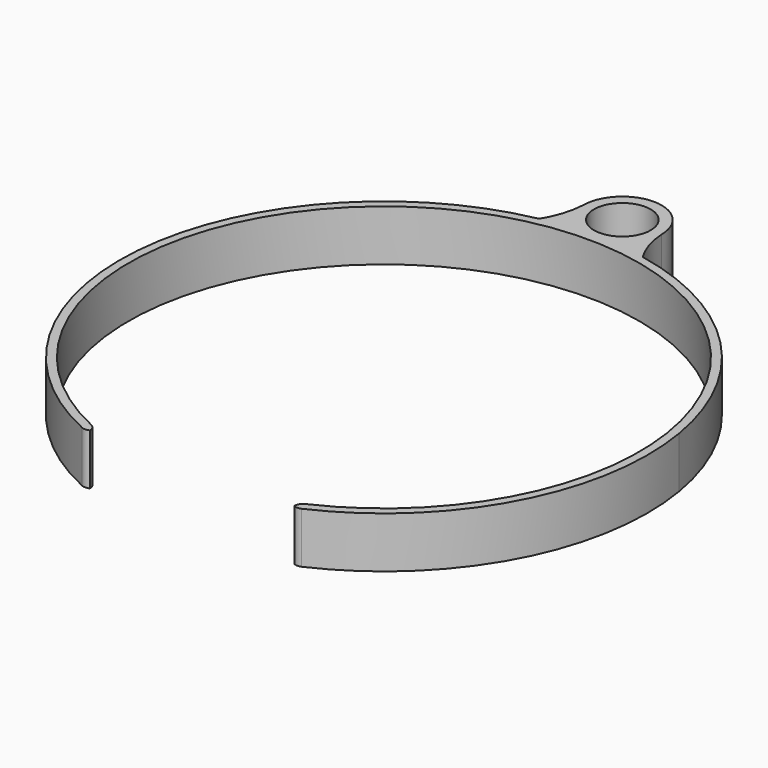
from build123d import *

# Parameters (mm, degrees)
F0_R         = 46.5
F0_R_2       = 45
F1_DEPTH     = 9
F3_DEPTH     = 25
F5_DEPTH     = 25
F7_DEPTH     = 9
F9_DEPTH     = 9
F11_DEPTH    = 9
F13_DEPTH    = 25
F15_DEPTH    = 25
F16_R        = 45
F17_DEPTH    = 9
F18_R        = 45
F19_DEPTH    = 25
F21_DEPTH    = 25
F22_R        = 1.55
F23_T1_DEPTH = 16.2900218994
F24_T1_DEPTH = 16.2900218994


# Not quite as in the source:
# - a fillet or chamfer that OpenCascade refuses, or shapes differently, is made with other operations: its cross-section is extruded or revolved along the edge and cut away or added


with BuildPart() as f1:
    # F0 (on Top) → F1 (new body)
    with BuildSketch(Plane.XY):
        Circle(F0_R)
        Circle(F0_R_2, mode=Mode.SUBTRACT)
    extrude(amount=F1_DEPTH)

    # F2 (on face) → F3 (cut)
    with BuildSketch(Plane.XY.offset(9)):
        Polygon((64.8135244846, -21.5104352683), (0, -21.5104352683), (-51.5724048018, -21.5104352683), (-51.5724048018, -59.9158406258), (64.033716917, -57.7713772655), align=None)
    extrude(amount=-F3_DEPTH, mode=Mode.SUBTRACT)

    # F4 (on face) → F5 (cut)
    with BuildSketch(Plane.XY.offset(9)):
        with BuildLine():
            ThreePointArc((-40.5525222975, -19.506228116), (-40.9032938672, -20.5072072896), (-41.9042730407, -20.1564357199))
            Line((-41.9042730407, -20.1564357199), (-43.4346050024, -22.7221362293))
            Line((-43.4346050024, -22.7221362293), (-36.3525599241, -23.4547629952))
            Line((-36.3525599241, -23.4547629952), (-40.5525222975, -19.506228116))
        make_face()
        with BuildLine():
            Line((43.4346050024, -22.7221362293), (41.9042730407, -20.1564357199))
            ThreePointArc((41.9042730407, -20.1564357199), (40.9032938672, -20.5072072896), (40.5525222975, -19.506228116))
            Line((40.5525222975, -19.506228116), (36.3525599241, -23.4547629952))
            Line((36.3525599241, -23.4547629952), (43.4346050024, -22.7221362293))
        make_face()
    extrude(amount=-F5_DEPTH, mode=Mode.SUBTRACT)

    # F6 (on face) → F7 (join)
    with BuildSketch(Plane.XY.offset(9)):
        with BuildLine():
            ThreePointArc((6.9320949163, 52.5), (-4.9017313232, 57.4017313232), (0, 45.5679050837))
            ThreePointArc((0, 45.5679050837), (4.9017313232, 47.5982686768), (6.9320949163, 52.5))
        make_face()
        with BuildLine():
            ThreePointArc((5, 52.5), (3.5355339059, 48.9644660941), (0, 47.5))
            ThreePointArc((0, 47.5), (-3.5355339059, 56.0355339059), (5, 52.5))
        make_face(mode=Mode.SUBTRACT)
    extrude(amount=-F7_DEPTH)

    # F8 (on face) → F9 (join)
    with BuildSketch(Plane.XY.offset(9)):
        with BuildLine():
            ThreePointArc((-6.9320949163, 52.5), (-7.6007884485, 48.9142518774), (-9.1181185374, 45.5972577502))
            ThreePointArc((-9.1181185374, 45.5972577502), (0, 45.60976302), (9.1181185374, 45.5972577502))
            ThreePointArc((9.1181185374, 45.5972577502), (7.6007884485, 48.9142518774), (6.9320949163, 52.5))
            ThreePointArc((6.9320949163, 52.5), (0, 47.0015761941), (-6.9320949163, 52.5))
        make_face()
    extrude(amount=-F9_DEPTH)

    # F10 (on face) → F11 (join)
    with BuildSketch(Plane.XY.offset(9)):
        with BuildLine():
            Line((-44.8310511788, 3.895747708), (-46.3451584316, 3.7916078319))
            ThreePointArc((-46.3451584316, 3.7916078319), (-42.7926175487, -9.5215818837), (-33.8443815708, -19.9996847659))
            ThreePointArc((-33.8443815708, -19.9996847659), (-32.8631083129, -20.2138563114), (-32.1503467858, -19.506228116))
            ThreePointArc((-32.1503467858, -19.506228116), (-41.2777702931, -9.315455738), (-44.8310511788, 3.895747708))
        make_face()
        with BuildLine():
            ThreePointArc((33.8443815708, -19.9996847659), (42.7926175487, -9.5215818837), (46.3451584316, 3.7916078319))
            Line((46.3451584316, 3.7916078319), (44.8310511788, 3.895747708))
            ThreePointArc((44.8310511788, 3.895747708), (41.2777702931, -9.315455738), (32.1503467858, -19.506228116))
            ThreePointArc((32.1503467858, -19.506228116), (32.8631083129, -20.2138563114), (33.8443815708, -19.9996847659))
        make_face()
    extrude(amount=-F11_DEPTH)

    # F12 (on face) → F13 (cut)
    with BuildSketch(Plane.XY.offset(9)):
        with BuildLine():
            ThreePointArc((-44.7172397739, -5.0367119241), (-45.830770977, -0.896267065), (-46.3787269492, 3.35614162))
            Line((-46.3787269492, 3.35614162), (-53.9689548314, -20.3920416534))
            Line((-53.9689548314, -20.3920416534), (-39.6306179464, -26.7084874213))
            Line((-39.6306179464, -26.7084874213), (-35.9670780599, -21.9711512327))
            Line((-35.9670780599, -21.9711512327), (-43.2941578329, -10.1593965665))
            Line((-43.2941578329, -10.1593965665), (-44.7172397739, -5.0367119241))
        make_face()
        with BuildLine():
            Line((53.9689548314, -20.3920416534), (46.3787269492, 3.35614162))
            ThreePointArc((46.3787269492, 3.35614162), (45.830770977, -0.896267065), (44.7172397739, -5.0367119241))
            Line((44.7172397739, -5.0367119241), (43.2941578329, -10.1593965665))
            Line((43.2941578329, -10.1593965665), (35.9670780599, -21.9711512327))
            Line((35.9670780599, -21.9711512327), (39.6306179464, -26.7084874213))
            Line((39.6306179464, -26.7084874213), (53.9689548314, -20.3920416534))
        make_face()
    extrude(amount=-F13_DEPTH, mode=Mode.SUBTRACT)

    # F14 (on face) → F15 (cut)
    with BuildSketch(Plane.XY.offset(9)):
        with BuildLine():
            ThreePointArc((-45.7581778434, -1.2523031469), (-46.1397679432, 3.2286956321), (-45.8552008738, 7.7169004675))
            ThreePointArc((-45.8552008738, 7.7169004675), (-48.5264373147, 3.20287819), (-45.7581778434, -1.2523031469))
        make_face()
        with BuildLine():
            ThreePointArc((45.7581778434, -1.2523031469), (48.5264373147, 3.20287819), (45.8552008738, 7.7169004675))
            ThreePointArc((45.8552008738, 7.7169004675), (46.1397679432, 3.2286956321), (45.7581778434, -1.2523031469))
        make_face()
    extrude(amount=-F15_DEPTH, mode=Mode.SUBTRACT)

    # F16 (on face) → F17 (join)
    with BuildSketch(Plane.XY.offset(9)):
        with BuildLine():
            ThreePointArc((-9.1181185374, 45.5972577502), (0, -46.5), (9.1181185374, 45.5972577502))
            ThreePointArc((9.1181185374, 45.5972577502), (0, 46.5), (-9.1181185374, 45.5972577502))
        make_face()
        Circle(F16_R, mode=Mode.SUBTRACT)
    extrude(amount=-F17_DEPTH)

    # F18 (on face) → F19 (cut)
    with BuildSketch(Plane.XY.offset(9)):
        Circle(F18_R)
    extrude(amount=-F19_DEPTH, mode=Mode.SUBTRACT)

    # F20 (on face) → F21 (cut)
    with BuildSketch(Plane.XY.offset(9)):
        Polygon((18, 0), (0, 0), (-18, 0), (-18, -69.9843019247), (18, -69.3941116333), align=None)
    extrude(amount=-F21_DEPTH, mode=Mode.SUBTRACT)

    # F22
    f22_edges = [f1.edges().sort_by_distance(p)[0] for p in [
        (-18, -41.243181, 4.5),
        (18, -41.243181, 4.5),
    ]]
    fillet(f22_edges, radius=F22_R)

    # F23: fillet of radius 1.5 on 1 edges, made by hand

    # F23_s2 → F23_t1 (cut)
    with BuildSketch(Plane.XY.offset(-3.6450109497)):
        with BuildLine():
            ThreePointArc((18, -42.2457098414), (18.6625262969, -42.4244445619), (19.3353236307, -42.2894225557))
            ThreePointArc((19.3353236307, -42.2894225557), (18.6699563348, -42.5873541143), (18, -42.8748177839))
            Line((18, -42.8748177839), (18, -42.2457098414))
        make_face()
    extrude(amount=F23_T1_DEPTH, mode=Mode.SUBTRACT)

    # F24: fillet of radius 1.5 on 1 edges, made by hand

    # F24_s2 → F24_t1 (cut)
    with BuildSketch(Plane.XY.offset(-3.6450109497)):
        with BuildLine():
            ThreePointArc((-18, -42.2457098414), (-18.6625262969, -42.4244445619), (-19.3353236307, -42.2894225557))
            ThreePointArc((-19.3353236307, -42.2894225557), (-18.6699563348, -42.5873541143), (-18, -42.8748177839))
            Line((-18, -42.8748177839), (-18, -42.2457098414))
        make_face()
    extrude(amount=F24_T1_DEPTH, mode=Mode.SUBTRACT)


solid = f1.part
